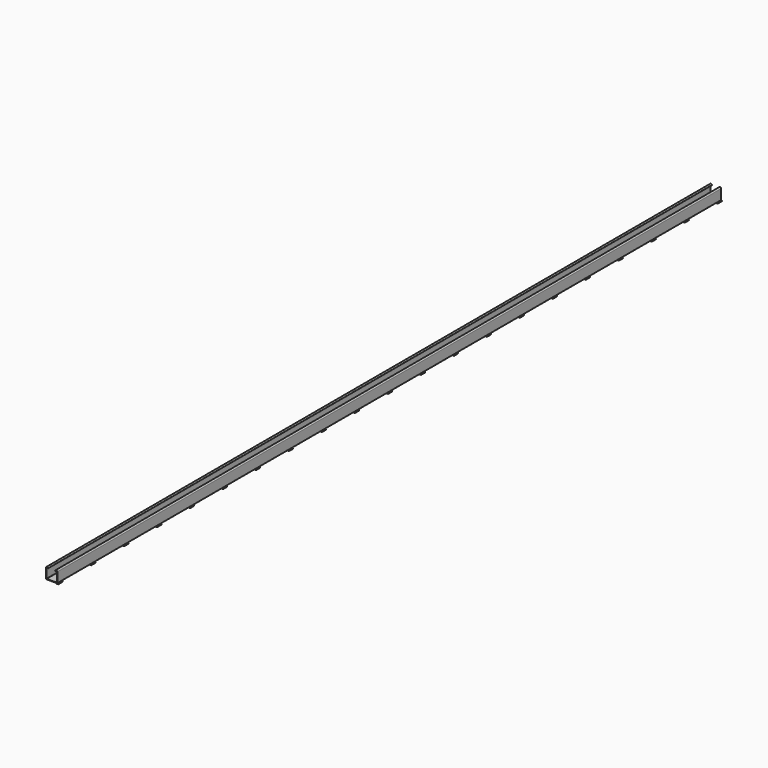
from build123d import *

# Parameters (mm, degrees)
F1_DEPTH = 1524
F2_R     = 0.79374
F3_W     = 19.05
F3_H     = 2.524125
F4_DEPTH = 3.175
F5_DEPTH = 2.38125


# Not quite as in the source:
# - a fillet or chamfer is up to 0.001 mm smaller than in the source, because OpenCascade refuses the exact size


with BuildPart() as f1:
    # F0 (on Front) → F1 (new body, symmetric)
    with BuildSketch(Plane.XZ):
        with BuildLine():
            Line((-20.6375, -20.6375), (20.6375, -20.6375))
            Line((20.6375, -20.6375), (20.6375, 16.6751))
            ThreePointArc((20.6375, 16.6751), (16.6751, 20.6375), (12.7127, 16.6751))
            Line((12.7127, 16.6751), (14.3002, 16.6751))
            ThreePointArc((14.3002, 16.6751), (16.6751, 19.05), (19.05, 16.6751))
            Line((19.05, 16.6751), (19.05, -19.05))
            Line((19.05, -19.05), (-19.05, -19.05))
            Line((-19.05, -19.05), (-19.05, 16.6751))
            ThreePointArc((-19.05, 16.6751), (-16.6751, 19.05), (-14.3002, 16.6751))
            Line((-14.3002, 16.6751), (-12.7127, 16.6751))
            ThreePointArc((-12.7127, 16.6751), (-16.6751, 20.6375), (-20.6375, 16.6751))
            Line((-20.6375, 16.6751), (-20.6375, -20.6375))
        make_face()
    extrude(amount=F1_DEPTH, both=True)

    # F2 (radius 0.79375 in the source; OpenCascade refuses exactly that, so slightly less here)
    f2_edges = [f1.edges().sort_by_distance(p)[0] for p in [
        (-20.6375, 0, -20.6375),
        (20.6375, 0, -20.6375),
        (-19.05, 0, -19.05),
        (19.05, 0, -19.05),
        (14.3002, 0, 16.6751),
        (12.7127, 0, 16.6751),
        (-14.3002, 0, 16.6751),
        (-12.7127, 0, 16.6751),
    ]]
    fillet(f2_edges, radius=F2_R)


with BuildPart() as f4:
    # F3 (on face) → F4 (new body)
    with BuildSketch(Plane.YZ.offset(20.6375)):
        with Locations((-1514.475, -21.7566875)):
            Rectangle(F3_W, F3_H)
    extrude(amount=F4_DEPTH)


with BuildPart() as f4b:
    # F3 (on face) → F4, piece 2 (new body)
    with BuildSketch(Plane.YZ.offset(20.6375)):
        with Locations((-1363.0275, -21.7566875)):
            Rectangle(F3_W, F3_H)
    extrude(amount=F4_DEPTH)


with BuildPart() as f4c:
    # F3 (on face) → F4, piece 3 (new body)
    with BuildSketch(Plane.YZ.offset(20.6375)):
        with Locations((-1211.58, -21.7566875)):
            Rectangle(F3_W, F3_H)
    extrude(amount=F4_DEPTH)


with BuildPart() as f4d:
    # F3 (on face) → F4, piece 4 (new body)
    with BuildSketch(Plane.YZ.offset(20.6375)):
        with Locations((-1060.1325, -21.7566875)):
            Rectangle(F3_W, F3_H)
    extrude(amount=F4_DEPTH)


with BuildPart() as f4e:
    # F3 (on face) → F4, piece 5 (new body)
    with BuildSketch(Plane.YZ.offset(20.6375)):
        with Locations((-908.685, -21.7566875)):
            Rectangle(F3_W, F3_H)
    extrude(amount=F4_DEPTH)


with BuildPart() as f4f:
    # F3 (on face) → F4, piece 6 (new body)
    with BuildSketch(Plane.YZ.offset(20.6375)):
        with Locations((-757.2375, -21.7566875)):
            Rectangle(F3_W, F3_H)
    extrude(amount=F4_DEPTH)


with BuildPart() as f4g:
    # F3 (on face) → F4, piece 7 (new body)
    with BuildSketch(Plane.YZ.offset(20.6375)):
        with Locations((-605.79, -21.7566875)):
            Rectangle(F3_W, F3_H)
    extrude(amount=F4_DEPTH)


with BuildPart() as f4h:
    # F3 (on face) → F4, piece 8 (new body)
    with BuildSketch(Plane.YZ.offset(20.6375)):
        with Locations((-454.3425, -21.7566875)):
            Rectangle(F3_W, F3_H)
    extrude(amount=F4_DEPTH)


with BuildPart() as f4i:
    # F3 (on face) → F4, piece 9 (new body)
    with BuildSketch(Plane.YZ.offset(20.6375)):
        with Locations((-302.895, -21.7566875)):
            Rectangle(F3_W, F3_H)
    extrude(amount=F4_DEPTH)


with BuildPart() as f4j:
    # F3 (on face) → F4, piece 10 (new body)
    with BuildSketch(Plane.YZ.offset(20.6375)):
        with Locations((-151.4475, -21.7566875)):
            Rectangle(F3_W, F3_H)
    extrude(amount=F4_DEPTH)


with BuildPart() as f4k:
    # F3 (on face) → F4, piece 11 (new body)
    with BuildSketch(Plane.YZ.offset(20.6375)):
        with Locations((0, -21.7566875)):
            Rectangle(F3_W, F3_H)
    extrude(amount=F4_DEPTH)


with BuildPart() as f4l:
    # F3 (on face) → F4, piece 12 (new body)
    with BuildSketch(Plane.YZ.offset(20.6375)):
        with Locations((151.4475, -21.7566875)):
            Rectangle(F3_W, F3_H)
    extrude(amount=F4_DEPTH)


with BuildPart() as f4m:
    # F3 (on face) → F4, piece 13 (new body)
    with BuildSketch(Plane.YZ.offset(20.6375)):
        with Locations((302.895, -21.7566875)):
            Rectangle(F3_W, F3_H)
    extrude(amount=F4_DEPTH)


with BuildPart() as f4n:
    # F3 (on face) → F4, piece 14 (new body)
    with BuildSketch(Plane.YZ.offset(20.6375)):
        with Locations((454.3425, -21.7566875)):
            Rectangle(F3_W, F3_H)
    extrude(amount=F4_DEPTH)


with BuildPart() as f4o:
    # F3 (on face) → F4, piece 15 (new body)
    with BuildSketch(Plane.YZ.offset(20.6375)):
        with Locations((605.79, -21.7566875)):
            Rectangle(F3_W, F3_H)
    extrude(amount=F4_DEPTH)


with BuildPart() as f4p:
    # F3 (on face) → F4, piece 16 (new body)
    with BuildSketch(Plane.YZ.offset(20.6375)):
        with Locations((757.2375, -21.7566875)):
            Rectangle(F3_W, F3_H)
    extrude(amount=F4_DEPTH)


with BuildPart() as f4q:
    # F3 (on face) → F4, piece 17 (new body)
    with BuildSketch(Plane.YZ.offset(20.6375)):
        with Locations((908.685, -21.7566875)):
            Rectangle(F3_W, F3_H)
    extrude(amount=F4_DEPTH)


with BuildPart() as f4r:
    # F3 (on face) → F4, piece 18 (new body)
    with BuildSketch(Plane.YZ.offset(20.6375)):
        with Locations((1060.1325, -21.7566875)):
            Rectangle(F3_W, F3_H)
    extrude(amount=F4_DEPTH)


with BuildPart() as f4s:
    # F3 (on face) → F4, piece 19 (new body)
    with BuildSketch(Plane.YZ.offset(20.6375)):
        with Locations((1211.58, -21.7566875)):
            Rectangle(F3_W, F3_H)
    extrude(amount=F4_DEPTH)


with BuildPart() as f4t:
    # F3 (on face) → F4, piece 20 (new body)
    with BuildSketch(Plane.YZ.offset(20.6375)):
        with Locations((1363.0275, -21.7566875)):
            Rectangle(F3_W, F3_H)
    extrude(amount=F4_DEPTH)


with BuildPart() as f4u:
    # F3 (on face) → F4, piece 21 (new body)
    with BuildSketch(Plane.YZ.offset(20.6375)):
        with Locations((1514.475, -21.7566875)):
            Rectangle(F3_W, F3_H)
    extrude(amount=F4_DEPTH)


with BuildPart() as f5:
    # F3 (on face) → F5 (new body)
    with BuildSketch(Plane.YZ.offset(20.6375)):
        with Locations((-1514.475, -21.7566875)):
            Rectangle(F3_W, F3_H)
    extrude(amount=-F5_DEPTH)


with BuildPart() as f5b:
    # F3 (on face) → F5, piece 2 (new body)
    with BuildSketch(Plane.YZ.offset(20.6375)):
        with Locations((-1363.0275, -21.7566875)):
            Rectangle(F3_W, F3_H)
    extrude(amount=-F5_DEPTH)


with BuildPart() as f5c:
    # F3 (on face) → F5, piece 3 (new body)
    with BuildSketch(Plane.YZ.offset(20.6375)):
        with Locations((-1211.58, -21.7566875)):
            Rectangle(F3_W, F3_H)
    extrude(amount=-F5_DEPTH)


with BuildPart() as f5d:
    # F3 (on face) → F5, piece 4 (new body)
    with BuildSketch(Plane.YZ.offset(20.6375)):
        with Locations((-1060.1325, -21.7566875)):
            Rectangle(F3_W, F3_H)
    extrude(amount=-F5_DEPTH)


with BuildPart() as f5e:
    # F3 (on face) → F5, piece 5 (new body)
    with BuildSketch(Plane.YZ.offset(20.6375)):
        with Locations((-908.685, -21.7566875)):
            Rectangle(F3_W, F3_H)
    extrude(amount=-F5_DEPTH)


with BuildPart() as f5f:
    # F3 (on face) → F5, piece 6 (new body)
    with BuildSketch(Plane.YZ.offset(20.6375)):
        with Locations((-757.2375, -21.7566875)):
            Rectangle(F3_W, F3_H)
    extrude(amount=-F5_DEPTH)


with BuildPart() as f5g:
    # F3 (on face) → F5, piece 7 (new body)
    with BuildSketch(Plane.YZ.offset(20.6375)):
        with Locations((-605.79, -21.7566875)):
            Rectangle(F3_W, F3_H)
    extrude(amount=-F5_DEPTH)


with BuildPart() as f5h:
    # F3 (on face) → F5, piece 8 (new body)
    with BuildSketch(Plane.YZ.offset(20.6375)):
        with Locations((-454.3425, -21.7566875)):
            Rectangle(F3_W, F3_H)
    extrude(amount=-F5_DEPTH)


with BuildPart() as f5i:
    # F3 (on face) → F5, piece 9 (new body)
    with BuildSketch(Plane.YZ.offset(20.6375)):
        with Locations((-302.895, -21.7566875)):
            Rectangle(F3_W, F3_H)
    extrude(amount=-F5_DEPTH)


with BuildPart() as f5j:
    # F3 (on face) → F5, piece 10 (new body)
    with BuildSketch(Plane.YZ.offset(20.6375)):
        with Locations((-151.4475, -21.7566875)):
            Rectangle(F3_W, F3_H)
    extrude(amount=-F5_DEPTH)


with BuildPart() as f5k:
    # F3 (on face) → F5, piece 11 (new body)
    with BuildSketch(Plane.YZ.offset(20.6375)):
        with Locations((0, -21.7566875)):
            Rectangle(F3_W, F3_H)
    extrude(amount=-F5_DEPTH)


with BuildPart() as f5l:
    # F3 (on face) → F5, piece 12 (new body)
    with BuildSketch(Plane.YZ.offset(20.6375)):
        with Locations((151.4475, -21.7566875)):
            Rectangle(F3_W, F3_H)
    extrude(amount=-F5_DEPTH)


with BuildPart() as f5m:
    # F3 (on face) → F5, piece 13 (new body)
    with BuildSketch(Plane.YZ.offset(20.6375)):
        with Locations((302.895, -21.7566875)):
            Rectangle(F3_W, F3_H)
    extrude(amount=-F5_DEPTH)


with BuildPart() as f5n:
    # F3 (on face) → F5, piece 14 (new body)
    with BuildSketch(Plane.YZ.offset(20.6375)):
        with Locations((454.3425, -21.7566875)):
            Rectangle(F3_W, F3_H)
    extrude(amount=-F5_DEPTH)


with BuildPart() as f5o:
    # F3 (on face) → F5, piece 15 (new body)
    with BuildSketch(Plane.YZ.offset(20.6375)):
        with Locations((605.79, -21.7566875)):
            Rectangle(F3_W, F3_H)
    extrude(amount=-F5_DEPTH)


with BuildPart() as f5p:
    # F3 (on face) → F5, piece 16 (new body)
    with BuildSketch(Plane.YZ.offset(20.6375)):
        with Locations((757.2375, -21.7566875)):
            Rectangle(F3_W, F3_H)
    extrude(amount=-F5_DEPTH)


with BuildPart() as f5q:
    # F3 (on face) → F5, piece 17 (new body)
    with BuildSketch(Plane.YZ.offset(20.6375)):
        with Locations((1060.1325, -21.7566875)):
            Rectangle(F3_W, F3_H)
    extrude(amount=-F5_DEPTH)


with BuildPart() as f5r:
    # F3 (on face) → F5, piece 18 (new body)
    with BuildSketch(Plane.YZ.offset(20.6375)):
        with Locations((908.685, -21.7566875)):
            Rectangle(F3_W, F3_H)
    extrude(amount=-F5_DEPTH)


with BuildPart() as f5s:
    # F3 (on face) → F5, piece 19 (new body)
    with BuildSketch(Plane.YZ.offset(20.6375)):
        with Locations((1211.58, -21.7566875)):
            Rectangle(F3_W, F3_H)
    extrude(amount=-F5_DEPTH)


with BuildPart() as f5t:
    # F3 (on face) → F5, piece 20 (new body)
    with BuildSketch(Plane.YZ.offset(20.6375)):
        with Locations((1363.0275, -21.7566875)):
            Rectangle(F3_W, F3_H)
    extrude(amount=-F5_DEPTH)


with BuildPart() as f5u:
    # F3 (on face) → F5, piece 21 (new body)
    with BuildSketch(Plane.YZ.offset(20.6375)):
        with Locations((1514.475, -21.7566875)):
            Rectangle(F3_W, F3_H)
    extrude(amount=-F5_DEPTH)


solid = Compound([f1.part, f4.part, f4b.part, f4c.part, f4d.part, f4e.part, f4f.part, f4g.part, f4h.part, f4i.part, f4j.part, f4k.part, f4l.part, f4m.part, f4n.part, f4o.part, f4p.part, f4q.part, f4r.part, f4s.part, f4t.part, f4u.part, f5.part, f5b.part, f5c.part, f5d.part, f5e.part, f5f.part, f5g.part, f5h.part, f5i.part, f5j.part, f5k.part, f5l.part, f5m.part, f5n.part, f5o.part, f5p.part, f5q.part, f5r.part, f5s.part, f5t.part, f5u.part])
